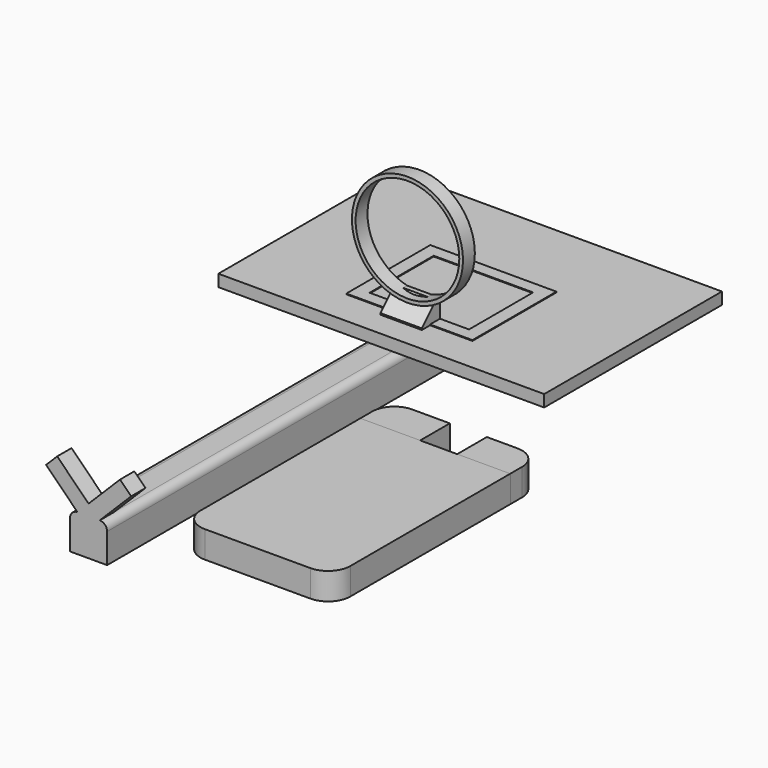
from build123d import *

# Parameters (mm, degrees)
F0_W          = 6.35
F0_H          = 6.35
F1_DEPTH      = 81.788
F2_R          = 1.27
F3_W          = 55.88
F3_H          = 38.1
F4_DEPTH      = 2.032
F5_W          = 21.6265805066
F5_H          = 17.9995894432
F5_W_2        = 17.0448683202
F5_H_2        = 13.7451440096
F6_DEPTH      = 0.127
F7_W          = 7.0821573026
F7_H          = 3.8917660713
F8_DEPTH      = 0.762
F9_W          = 7.0821573026
F9_H          = 3.8917660713
F10_DEPTH     = 2.54
F11_SIZE      = 3.048
F14_R         = 9.525
F14_R_2       = 8.89
F15_DEPTH     = 2.54
F16_W         = 3.81
F16_H         = 3.0767128337
F17_DEPTH     = 2.54
F18_T4_DEPTH  = 16.1408624126
F18_S5_R      = 1.27
F18_T6_DEPTH  = 10
F18_T10_DEPTH = 16.1408624126
F18_S11_R     = 1.27
F18_T12_DEPTH = 10
F19_DEPTH     = 7.62
F21_W         = 2.6957672939
F21_H         = 3.0767128337
F22_DEPTH     = 7.62
F23_W         = 25.7097072899
F23_H         = 4.6064495109
F24_DEPTH     = 38.1
F25_DEPTH     = 6.35
F26_R         = 3.81
F26_2_R       = 3.81
F27_W         = 6.35
F27_H         = 4.6923138624
F28_DEPTH     = 6.35
F29_ANGLE     = 90
F30_ANGLE     = 270


# Not quite as in the source:
# - a fillet or chamfer that OpenCascade refuses, or shapes differently, is made with other operations: its cross-section is extruded or revolved along the edge and cut away or added
# - a feature of the source that left no trace in its solid (it failed there, or was rolled back) is left out


with BuildPart() as f1:
    # F0 (on Top) → F1 (new body)
    with BuildSketch(Plane.XY):
        Rectangle(F0_W, F0_H)
    extrude(amount=F1_DEPTH)

    # F2
    f2_edges = [f1.edges().sort_by_distance(p)[0] for p in [
        (-3.175, -3.175, 40.894),
        (3.175, -3.175, 40.894),
    ]]
    fillet(f2_edges, radius=F2_R)

    # F3 (on face) → F4 (join)
    with BuildSketch(Plane.XZ.offset(3.175)):
        with Locations((0, 81.788)):
            Rectangle(F3_W, F3_H)
    extrude(amount=F4_DEPTH)

    # F5 (on face) → F6 (join)
    with BuildSketch(Plane.XZ.offset(5.207)):
        with Locations((0, 77.7648165822)):
            Rectangle(F5_W, F5_H)
        with Locations((0, 77.7648165822)):
            Rectangle(F5_W_2, F5_H_2, mode=Mode.SUBTRACT)
    extrude(amount=F6_DEPTH)

    # F7 (on face) → F8 (join)
    with BuildSketch(Plane.XZ.offset(5.207)):
        with Locations((0, 68.9463615417)):
            Rectangle(F7_W, F7_H)
    extrude(amount=F8_DEPTH)

    # F9 (on face) → F10 (join)
    with BuildSketch(Plane.XZ.offset(5.969)):
        with Locations((0, 68.9463615417)):
            Rectangle(F9_W, F9_H)
    extrude(amount=F10_DEPTH)

    # F11
    f11_edges = [f1.edges().sort_by_distance(p)[0] for p in [
        (0, -8.509, 67.000479),
    ]]
    chamfer(f11_edges, length=F11_SIZE)

    # F14 (on face) → F15 (join)
    with BuildSketch(Plane.XY.offset(70.8922445774)):
        with Locations((0, -17.1449985355)):
            Circle(F14_R)
        with Locations((0, -17.1449985355)):
            Circle(F14_R_2, mode=Mode.SUBTRACT)
    extrude(amount=-F15_DEPTH)

    # F16 (on face) → F17 (join)
    with BuildSketch(Plane.XZ.offset(3.175)):
        with Locations((0, 1.5383564169)):
            Rectangle(F16_W, F16_H)
    extrude(amount=F17_DEPTH)

    # F18: chamfer of 2.54 on 2 edges, made by hand


with BuildPart() as f18_tool2:
    # F18_s3 → F18_t4 (new body)
    with BuildSketch(Plane.XY.offset(-6.5320747894)):
        Polygon((1.905, -3.175), (-0.635, -5.715), (1.905, -5.715), align=None)
    extrude(amount=F18_T4_DEPTH)

    # F18_s5 → F18_t6 (cut, symmetric)
    with BuildSketch(Plane.XY.offset(1.5)):
        with Locations((1.905, -1.905)):
            Circle(F18_S5_R)
    extrude(amount=F18_T6_DEPTH, both=True, mode=Mode.SUBTRACT)


with BuildPart() as f1_1:
    add(f1.part)

    # F18_t1: cut F18_tool2
    add(f18_tool2.part, mode=Mode.SUBTRACT)


with BuildPart() as f18_tool8:
    # F18_s9 → F18_t10 (new body)
    with BuildSketch(Plane.XY.offset(9.6087876232)):
        Polygon((-1.905, -3.175), (0.635, -5.715), (-1.905, -5.715), align=None)
    extrude(amount=-F18_T10_DEPTH)

    # F18_s11 → F18_t12 (cut, symmetric)
    with BuildSketch(Plane.XY.offset(1.5)):
        with Locations((-1.905, -1.905)):
            Circle(F18_S11_R)
    extrude(amount=F18_T12_DEPTH, both=True, mode=Mode.SUBTRACT)


with BuildPart() as f1_2:
    add(f1_1.part)

    # F18_t7: cut F18_tool8
    add(f18_tool8.part, mode=Mode.SUBTRACT)

    # F19 (add): a face of the model
    f19_faces = [f1_2.faces().sort_by_distance(p)[0] for p in [
        (-0.9525, -4.1275, 1.5383564169),
    ]]
    extrude(f19_faces, amount=F19_DEPTH)

    # F21 (on face) → F22 (join)
    with BuildSketch(Plane(origin=(2.54, -2.54, 0), x_dir=(0.7071067812, 0.7071067812, 0), z_dir=(0.7071067812, -0.7071067812, 0))):
        with Locations((-2.2459092591, 1.5383564169)):
            Rectangle(F21_W, F21_H)
    extrude(amount=F22_DEPTH)


with BuildPart() as f24:
    # F23 (on face) → F24 (new body)
    with BuildSketch(Plane.YZ):
        with Locations((-47.2440104932, 2.3032247555)):
            Rectangle(F23_W, F23_H)
    extrude(amount=F24_DEPTH)


with BuildPart() as f25:
    # F25 (new): faces of the model
    f25_faces = [f24.part.faces().sort_by_distance(p)[0] for p in [
        (0, -47.2440104932, 2.3032247555),
        (0, -47.2440104932, 2.3032247555),
    ]]
    extrude(f25_faces, amount=F25_DEPTH)

    # F26#2
    f26_2_edges = [f25.edges().sort_by_distance(p)[0] for p in [
        (-6.35, -34.389157, 2.303225),
        (-6.35, -60.098864, 2.303225),
    ]]
    fillet(f26_2_edges, radius=F26_2_R)

    # F27 (on face) → F28 (cut)
    with BuildSketch(Plane(origin=(-6.35, 0, 0), x_dir=(0, -1, 0), z_dir=(-1, 0, 0))):
        with Locations((46.6604062438, 2.3461569312)):
            Rectangle(F27_W, F27_H)
    extrude(amount=-F28_DEPTH, mode=Mode.SUBTRACT)


with BuildPart() as f24_1:
    add(f24.part)

    # F26
    f26_edges = [f24_1.edges().sort_by_distance(p)[0] for p in [
        (38.1, -34.389157, 2.303225),
        (38.1, -60.098864, 2.303225),
    ]]
    fillet(f26_edges, radius=F26_R)


with BuildPart() as f1_3:
    # F29: moved
    add(f1_2.part.rotate(Axis((0, 3.175, 0), (-1, 0, 0)), F29_ANGLE))


with BuildPart() as f24_2:
    # F30: moved
    add(f24_1.part.rotate(Axis((34.29, -34.3891568482, 2.3032247555), (0, 0, 1)), F30_ANGLE))


with BuildPart() as f25_1:
    # F30: moved
    add(f25.part.rotate(Axis((34.29, -34.3891568482, 2.3032247555), (0, 0, 1)), F30_ANGLE))


with BuildPart() as f1_4:
    # F31: moved
    add(f1_3.part.moved(Location((0, -50.8, 0))))


solid = Compound([f24_2.part, f25_1.part, f1_4.part])
